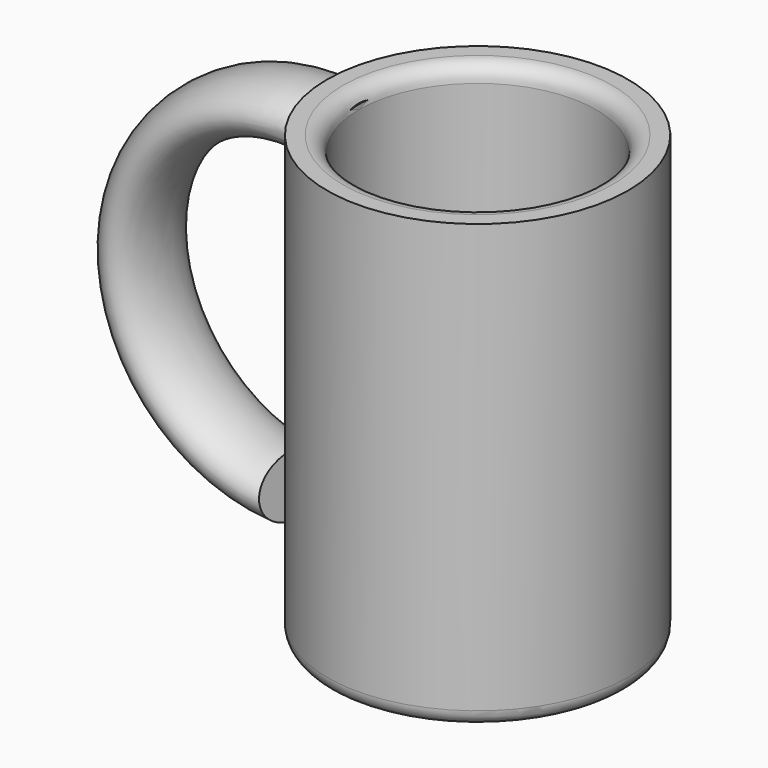
from build123d import *

# Parameters (mm, degrees)
F2_R = 3


with BuildPart() as f1:
    # F0 (on Front) → F1 (revolve)
    with BuildSketch(Plane.XZ):
        Polygon((-27.94, 0), (0, 0), (0, 7), (-22, 7), (-22, 82.55), (-27.94, 82.55), align=None)
    revolve(axis=Axis((0, 0, 3.5), (0, 0, -1)))

    # F2
    f2_edges = [f1.edges().sort_by_distance(p)[0] for p in [
        (22, 0, 82.55),
        (27.94, 0, 0),
    ]]
    fillet(f2_edges, radius=F2_R)

    # F6: sweep along a path in F4
    with BuildLine(Plane.XZ) as f6_path:
        ThreePointArc((-27.9568824917, 75.0939920545), (-60.8796643301, 45.6174495611), (-28.1154159456, 15.9647911787))
    # F5 (on line) → F6 (sweep)
    with BuildSketch(Plane(origin=(-22, 0, 0), x_dir=(0, -1, 0), z_dir=(-1, 0, 0))):
        with BuildLine():
            add(Edge.make_bspline(
                [(8.2423, 75.3380134702), (8.2423, 84.1801954249), (-4.12115, 79.7591044475), (-16.4846, 75.3380134702), (-4.12115, 70.9169224928), (8.2423, 66.4958315155), (8.2423, 75.3380134702)],
                knots=[0, 0, 0, 2.0943951024, 2.0943951024, 4.1887902048, 4.1887902048, 6.2831853072, 6.2831853072, 6.2831853072], degree=2, weights=[1, 0.5, 1, 0.5, 1, 0.5, 1]))
        make_face()
    sweep(path=f6_path.line)


solid = f1.part
